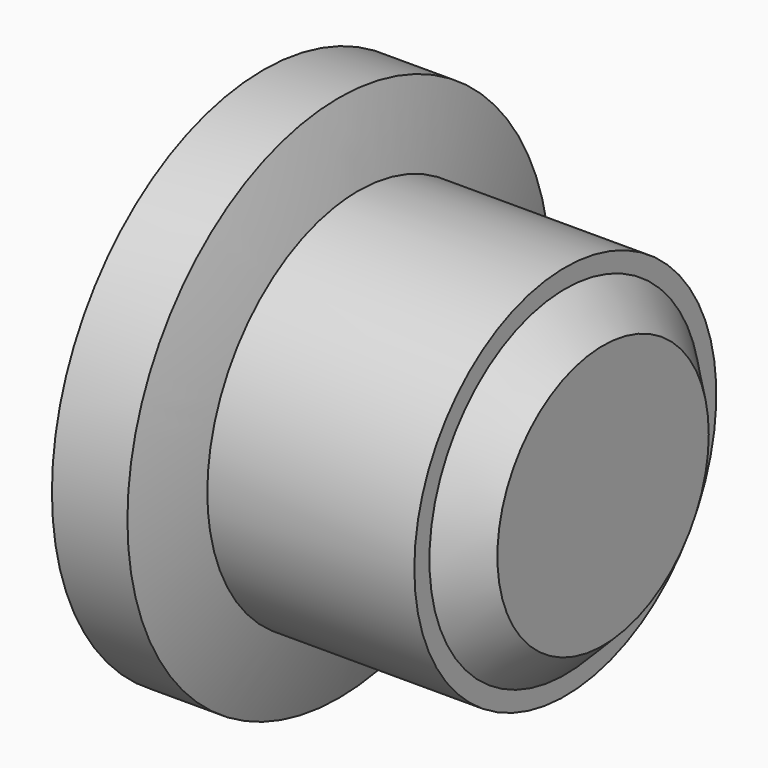
from build123d import *

# Parameters (mm, degrees)
F2_R     = 5
F3_DEPTH = 8
F4_R     = 4.5
F5_DEPTH = 1
F6_SIZE  = 0.99999


# Not quite as in the source:
# - a fillet or chamfer is up to 0.001 mm smaller than in the source, because OpenCascade refuses the exact size


with BuildPart() as f1:
    # F0 (on Front) → F1 (revolve)
    with BuildSketch(Plane.XZ):
        with BuildLine():
            Line((-3.0435194335, 0), (0, 0))
            ThreePointArc((0, 0), (-0.2623133647, 3.5386767586), (-1.0435194335, 7))
            Line((-1.0435194335, 7), (-3.0435194335, 7))
            Line((-3.0435194335, 7), (-3.0435194335, 0))
        make_face()
    revolve(axis=Axis((-1.5217597168, 0, 0), (1, 0, 0)))

    # F2 (on face) → F3 (join)
    with BuildSketch(Plane(origin=(-3.0435194335, 0, 0), x_dir=(0, -1, 0), z_dir=(-1, 0, 0))):
        Circle(F2_R)
    extrude(amount=-F3_DEPTH)

    # F4 (on face) → F5 (join)
    with BuildSketch(Plane.YZ.offset(4.9564805665)):
        Circle(F4_R)
    extrude(amount=F5_DEPTH)

    # F6 (size 1 in the source; OpenCascade refuses exactly that, so slightly less here)
    f6_edges = [f1.edges().sort_by_distance(p)[0] for p in [
        (5.956481, -4.5, 0),
    ]]
    chamfer(f6_edges, length=F6_SIZE)


solid = f1.part
